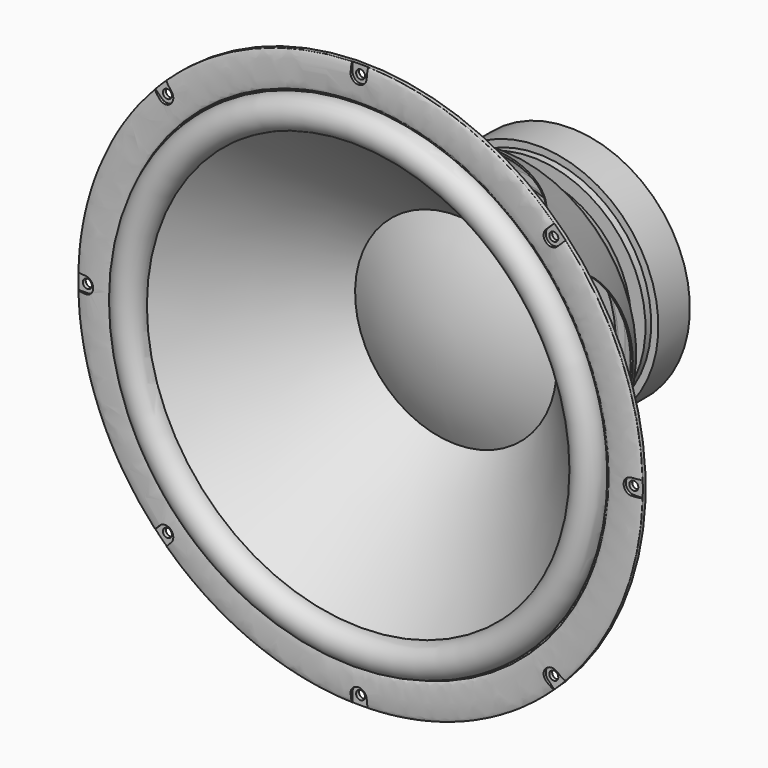
from build123d import *

# Parameters (mm, degrees)
F1_R            = 2.5
F4_DEPTH        = 3.5010001
F4_COPIES_COUNT = 8
F5_START        = 2
F5_DEPTH        = 1.5010001
F5_COPIES_COUNT = 8
F7_REACH        = 302.8196885229
F7_COPIES_COUNT = 4


# Not quite as in the source:
# - a pattern or mirror of a feature is missing from the dataset's text; its kind, count and spacing are read off the source's solid


with BuildPart() as f3:
    # F2 (on Top) → F3 (revolve)
    with BuildSketch(Plane.XY):
        with BuildLine():
            Line((-157.5, 0), (-157.5, -2))
            add(Edge.make_bspline(
                [(-157.5, -2), (-157.5, -4), (-138.5, -4), (-138.5, -2)],
                knots=[0, 0, 0, 0, 19, 19, 19, 19], degree=3))
            Line((-138.5, -2), (-138.5, 0))
            Line((-138.5, 0), (-157.5, 0))
        make_face()
        with BuildLine():
            Line((-138.5, 0), (-138.5, -2))
            Line((-138.5, -2), (-137.8, -2))
            ThreePointArc((-137.8, -2), (-137.5878679656, -1.9121320344), (-137.5, -1.7))
            Line((-137.5, -1.7), (-137.5, 0))
            Line((-137.5, 0), (-137.5, 13.7311574336))
            Line((-137.5, 13.7311574336), (-134.446312364, 19))
            Line((-134.446312364, 19), (-116.2383128768, 19))
            ThreePointArc((-116.2383128768, 19), (-114.6799972005, 19.436476594), (-113.5751270701, 20.6188984979))
            Line((-113.5751270701, 20.6188984979), (-75.4636018887, 94.1095671974))
            ThreePointArc((-75.4636018887, 94.1095671974), (-74.7571338128, 95.1950212532), (-73.8517576223, 96.1210890711))
            Line((-73.8517576223, 96.1210890711), (-72.5942651494, 97.1762505413))
            ThreePointArc((-72.5942651494, 97.1762505413), (-69.8873579522, 98.7390841403), (-66.8091766622, 99.2818505533))
            Line((-66.8091766622, 99.2818505533), (-62.8492940813, 99.2818505533))
            ThreePointArc((-62.8492940813, 99.2818505533), (-61.1285647723, 99.8243944204), (-60.030216219, 101.2557901233))
            Line((-60.030216219, 101.2557901233), (-53.9068869091, 118.0794991339))
            Line((-53.9068869091, 118.0794991339), (-4, 118.0794991339))
            Line((-4, 118.0794991339), (-4, 146))
            ThreePointArc((-4, 146), (-5.1715728753, 148.8284271247), (-8, 150))
            Line((-8, 150), (-56.7514036, 150))
            Line((-56.7514036, 150), (-60.2514036, 146.5))
            Line((-60.2514036, 146.5), (-60.2514036, 144))
            Line((-60.2514036, 144), (-67, 144))
            Line((-67, 144), (-67, 122))
            Line((-67, 122), (-63, 122))
            Line((-63, 122), (-63, 118))
            Line((-63, 118), (-55, 118))
            Line((-55, 118), (-60.9699088397, 101.5978102666))
            ThreePointArc((-60.9699088397, 101.5978102666), (-61.7021412086, 100.6435464647), (-62.8492940813, 100.2818505533))
            Line((-62.8492940813, 100.2818505533), (-66.8091766622, 100.2818505533))
            ThreePointArc((-66.8091766622, 100.2818505533), (-70.2293780955, 99.6787767611), (-73.2370527591, 97.9422949845))
            Line((-73.2370527591, 97.9422949845), (-74.494545232, 96.8871335142))
            ThreePointArc((-74.494545232, 96.8871335142), (-75.5375052744, 95.8203374789), (-76.3513304909, 94.5699343647))
            Line((-76.3513304909, 94.5699343647), (-114.4628556723, 21.0792656652))
            ThreePointArc((-114.4628556723, 21.0792656652), (-115.1994357593, 20.290984396), (-116.2383128768, 20))
            Line((-116.2383128768, 20), (-133.8700726846, 20))
            ThreePointArc((-133.8700726846, 20), (-134.8686289453, 19.732883549), (-135.6004544014, 19.0028853942))
            Line((-135.6004544014, 19.0028853942), (-138.2303817169, 14.4652002615))
            ThreePointArc((-138.2303817169, 14.4652002615), (-138.4314196118, 13.9815626724), (-138.5, 13.4623148673))
            Line((-138.5, 13.4623148673), (-138.5, 0))
        make_face()
    revolve(axis=Axis((0, 0, 0), (0, -1, 0)))

    # F1 (on Front) → F4 (cut, through all)
    with BuildSketch(Plane.XZ):
        with Locations((-152.5, 0)):
            Circle(F1_R)
    f4 = extrude(amount=F4_DEPTH, mode=Mode.SUBTRACT)

    # F4_copies: F4 ×8 about axis
    f4_copies_axis = Axis((0, 0, 0), (0, 1, 0))
    for i in range(1, F4_COPIES_COUNT):
        add(f4.rotate(f4_copies_axis, i * 360 / F4_COPIES_COUNT), mode=Mode.SUBTRACT)

    # F1 (on Front) → F5 (cut)
    with BuildSketch(Plane.XZ.offset(F5_START)):
        with BuildLine():
            Line((-157.5, 4.5), (-157.5, -4.5))
            Line((-157.5, -4.5), (-152.5, -4.5))
            ThreePointArc((-152.5, -4.5), (-148, 0), (-152.5, 4.5))
            Line((-152.5, 4.5), (-157.5, 4.5))
        make_face()
        with Locations((-152.5, 0)):
            Circle(F1_R, mode=Mode.SUBTRACT)
    f5 = extrude(amount=F5_DEPTH, mode=Mode.SUBTRACT)

    # F5_copies: F5 ×8 about axis
    f5_copies_axis = Axis((0, 0, 0), (0, 1, 0))
    for i in range(1, F5_COPIES_COUNT):
        add(f5.rotate(f5_copies_axis, i * 360 / F5_COPIES_COUNT), mode=Mode.SUBTRACT)

    f7_end = f3.faces().sort_by_distance((95.4070930816, 57.824600015, 0))[0]
    # F6 (on Right) → F7 (cut, up to a face of the model that its end follows)
    with BuildSketch(Plane.YZ):
        with BuildLine():
            Line((24.0028853942, 65.0934278965), (24.0028853942, -65.0934278965))
            ThreePointArc((24.0028853942, -65.0934278965), (88.5699343647, 0), (24.0028853942, 65.0934278965))
        make_face()
    f7_long = extrude(amount=-F7_REACH, mode=Mode.PRIVATE)
    f7 = split(f7_long, bisect_by=f7_end, keep=Keep.BOTTOM, mode=Mode.PRIVATE)
    add(f7, mode=Mode.SUBTRACT)

    # F7_copies: F7 ×4 about axis
    f7_copies_axis = Axis((0, 0, 0), (0, 1, 0))
    for i in range(1, F7_COPIES_COUNT):
        add(f7.rotate(f7_copies_axis, i * 360 / F7_COPIES_COUNT), mode=Mode.SUBTRACT)


with BuildPart() as f9:
    # F8 (on Right) → F9 (revolve)
    with BuildSketch(Plane.YZ):
        with BuildLine():
            Line((-1.7594667872, -120.1974694984), (-1.7, -119.5))
            ThreePointArc((-1.7, -119.5), (-11.5, -128.5), (-1.7, -137.5))
            Line((-1.7, -137.5), (-1.7594667872, -136.8025305016))
            ThreePointArc((-1.7594667872, -136.8025305016), (-10.8, -128.5), (-1.7594667872, -120.1974694984))
        make_face()
    revolve(axis=Axis((0, 0, 0), (0, -1, 0)))


with BuildPart() as f11:
    # F10 (on Right) → F11 (revolve)
    with BuildSketch(Plane.YZ):
        with BuildLine():
            Line((64.4957565326, -56.2757817263), (64.8718162922, -55.9166033503))
            ThreePointArc((64.8718162922, -55.9166033503), (54.5840952868, -28.7953351232), (51.0870867265, 0))
            Line((51.0870867265, 0), (50.5870867265, 0))
            ThreePointArc((50.5870867265, 0), (54.1157916861, -28.984542021), (64.4957565326, -56.2757817263))
        make_face()
    revolve(axis=Axis((0, 13.0399312973, 0), (0, -1, 0)))


with BuildPart() as f11b:
    # F10 (on Right) → F11, piece 2 (revolve)
    with BuildSketch(Plane.YZ):
        with BuildLine():
            Line((118, -20), (118, -19.5))
            Line((118, -19.5), (103, -19.5))
            Line((103, -19.5), (64.8718162922, -55.9166033503))
            ThreePointArc((64.8718162922, -55.9166033503), (64.9049838878, -55.9797403705), (64.938188907, -56.0428577169))
            Line((64.938188907, -56.0428577169), (64.4957565326, -56.2757817263))
            Line((64.4957565326, -56.2757817263), (-1.7, -119.5))
            Line((-1.7, -119.5), (-1.3546553649, -119.861575833))
            Line((-1.3546553649, -119.861575833), (103.2004145322, -20))
            Line((103.2004145322, -20), (118, -20))
        make_face()
    revolve(axis=Axis((0, 13.0399312973, 0), (0, -1, 0)))


solid = Compound([f3.part, f9.part, f11.part, f11b.part])
